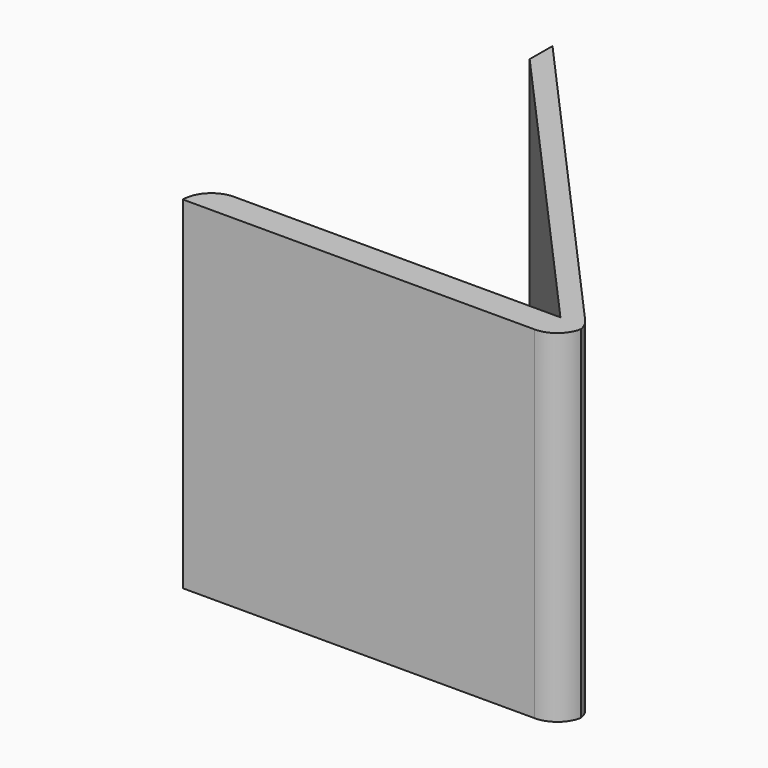
from build123d import *

# Parameters (mm, degrees)
F1_DEPTH    = 18
F2_T1_DEPTH = 25.5
F2_T3_DEPTH = 20.8647450844


# Not quite as in the source:
# - a fillet or chamfer that OpenCascade refuses, or shapes differently, is made with other operations: its cross-section is extruded or revolved along the edge and cut away or added


with BuildPart() as f1:
    # F0 (on Top) → F1 (new body)
    with BuildSketch(Plane.XY):
        Polygon((-16.1896759786, 48.2207899958), (-34.8480351921, 48.2207899958), (-34.8480351921, 46.7207899958), (-14.8480351921, 46.7207899958), (-14.8480351921, 48.2207899958), (-31.5147018588, 66.8546898083), (-31.523009312, 65.3639778233), align=None)
    extrude(amount=F1_DEPTH)

    # F2: fillet of radius 1.5 on 3 edges, made by hand

    # F2_s2 → F2_t1 (cut)
    with BuildSketch(Plane.XY.offset(-3.75)):
        with BuildLine():
            ThreePointArc((-16.3480351921, 46.7207899958), (-15.2873750203, 47.160129824), (-14.8480351921, 48.2207899958))
            Line((-14.8480351921, 48.2207899958), (-14.8480351921, 46.7207899958))
            Line((-14.8480351921, 46.7207899958), (-16.3480351921, 46.7207899958))
        make_face()
        with BuildLine():
            ThreePointArc((-33.3480351921, 48.2207899958), (-34.4086953639, 47.7814501676), (-34.8480351921, 46.7207899958))
            Line((-34.8480351921, 46.7207899958), (-34.8480351921, 48.2207899958))
            Line((-34.8480351921, 48.2207899958), (-33.3480351921, 48.2207899958))
        make_face()
    extrude(amount=F2_T1_DEPTH, mode=Mode.SUBTRACT)

    # F2_s4 → F2_t3 (cut)
    with BuildSketch(Plane.XY.offset(-1.4323725422)):
        with BuildLine():
            ThreePointArc((-14.8480351921, 47.6478409789), (-14.9467766537, 48.1830741136), (-15.2300012034, 48.6478409789))
            Line((-15.2300012034, 48.6478409789), (-14.8480351921, 48.2207899958))
            Line((-14.8480351921, 48.2207899958), (-14.8480351921, 47.6478409789))
        make_face()
    extrude(amount=F2_T3_DEPTH, mode=Mode.SUBTRACT)


solid = f1.part
